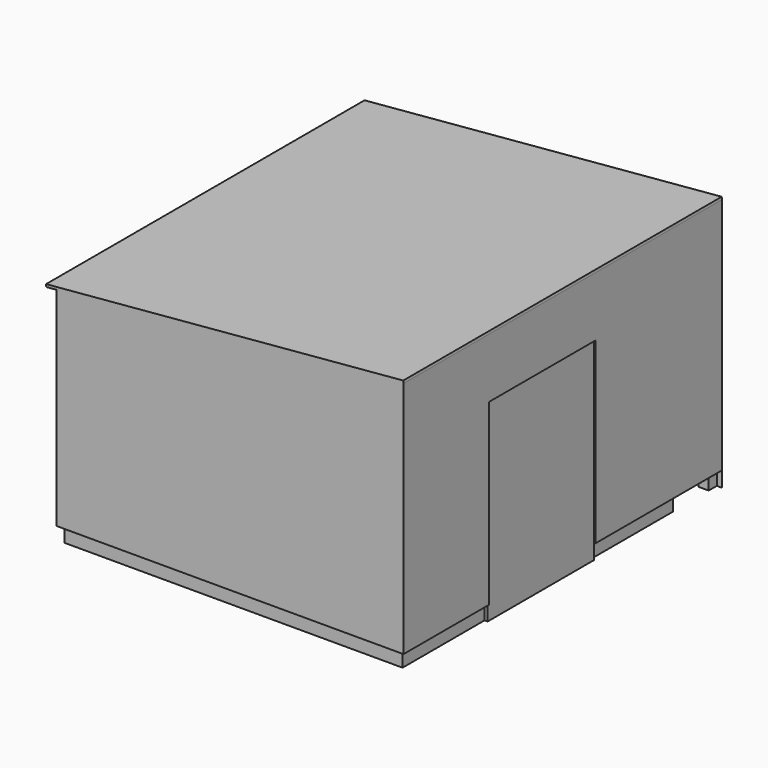
from build123d import *

# Parameters (mm, degrees)
F0_W      = 3300
F0_H      = 3300
F3_REACH  = 7658.4274260304
F4_W      = 3512.9874476474
F4_H      = 3900
F5_DEPTH  = 25
F0_W_2    = 100
F0_H_2    = 100
F8_DEPTH  = 15
F10_W     = 3400
F10_H     = 150
F11_DEPTH = 45
F9_W      = 3400
F9_H      = 150
F12_DEPTH = 45
F13_W     = 3305
F13_H     = 150
F14_DEPTH = 45
F7_W      = 1050
F7_H      = 150
F15_DEPTH = 45
F7_W_2    = 1004.8515605927
F16_DEPTH = 45
F7_W_3    = 545
F17_DEPTH = 50


with BuildPart() as f3:
    f3_end = Plane(origin=(-189.8836434212, 0, 2170.3799757433), x_dir=(0.9961946981, 0, 0.0871557427), z_dir=(-0.0871557427, 0, 0.9961946981))
    # F0 (on Top) → F3 (new body, up to a plane its end follows)
    with BuildSketch(Plane.XY):
        Polygon((0, 3400), (0, 0), (3400, 0), (3400, 3400), (3400, 3899.8515605927), (3350, 3900), (3350, 3800), (3350, 3400), align=None)
        with Locations((1700, 1700)):
            Rectangle(F0_W, F0_H, mode=Mode.SUBTRACT)
    f3_long = extrude(amount=F3_REACH, mode=Mode.PRIVATE)
    add(split(f3_long, bisect_by=f3_end, keep=Keep.BOTTOM, mode=Mode.PRIVATE))

    # F4 (on offset) → F5 (join)
    with BuildSketch(Plane(origin=(-189.8836434212, 0, 2170.3799757433), x_dir=(0.9961946981, 0, 0.0871557427), z_dir=(-0.0871557427, 0, 0.9961946981))):
        with Locations((1847.1026919149, 1950)):
            Rectangle(F4_W, F4_H)
    extrude(amount=F5_DEPTH)

    # F0 (on Top) → F6 (join, up to the next surface of F3)
    with BuildSketch(Plane.XY):
        with Locations((3300, 3850)):
            Rectangle(F0_W_2, F0_H_2)
    extrude(until=Until.NEXT)

    # F7 (on face) → F8 (cut)
    with BuildSketch(Plane.YZ.offset(3400)):
        Polygon((1450, 1900), (1450, 0), (2350, 0), (2350, 150), (2350, 275), (2350, 400), (2350, 525), (2350, 650), (2350, 775), (2350, 900), (2350, 1025), (2350, 1150), (2350, 1275), (2350, 1400), (2350, 1525), (2350, 1650), (2350, 1775), (2350, 1900), align=None)
        Polygon((1050, 150), (1050, 0), (1450, 0), (1450, 1900), (1050, 1900), (1050, 1775), (1050, 1650), (1050, 1525), (1050, 1400), (1050, 1275), (1050, 1150), (1050, 1025), (1050, 900), (1050, 775), (1050, 650), (1050, 525), (1050, 400), (1050, 275), align=None)
    extrude(amount=-F8_DEPTH, mode=Mode.SUBTRACT)

    # F10 (on face) → F11 (cut)
    with BuildSketch(Plane(origin=(0, 0, 0), x_dir=(0, -1, 0), z_dir=(-1, 0, 0))):
        with Locations((-1700, 75)):
            Rectangle(F10_W, F10_H)
    extrude(amount=-F11_DEPTH, mode=Mode.SUBTRACT)

    # F9 (on face) → F12 (cut)
    with BuildSketch(Plane.XZ):
        with Locations((1700, 75)):
            Rectangle(F9_W, F9_H)
    extrude(amount=-F12_DEPTH, mode=Mode.SUBTRACT)

    # F13 (on face) → F14 (cut)
    with BuildSketch(Plane(origin=(0, 3400, 0), x_dir=(-1, 0, 0), z_dir=(0, 1, 0))):
        with Locations((-1697.5, 75)):
            Rectangle(F13_W, F13_H)
    extrude(amount=-F14_DEPTH, mode=Mode.SUBTRACT)

    # F7 (on face) → F15 (cut)
    with BuildSketch(Plane.YZ.offset(3400)):
        with Locations((525, 75)):
            Rectangle(F7_W, F7_H)
    extrude(amount=-F15_DEPTH, mode=Mode.SUBTRACT)

    # F7 (on face) → F16 (cut)
    with BuildSketch(Plane.YZ.offset(3400)):
        with Locations((2852.4257802963, 75)):
            Rectangle(F7_W_2, F7_H)
    extrude(amount=-F16_DEPTH, mode=Mode.SUBTRACT)

    # F7 (on face) → F17 (cut)
    with BuildSketch(Plane.YZ.offset(3400)):
        with Locations((3627.3515605927, 75)):
            Rectangle(F7_W_3, F7_H)
    extrude(amount=-F17_DEPTH, mode=Mode.SUBTRACT)


solid = f3.part
